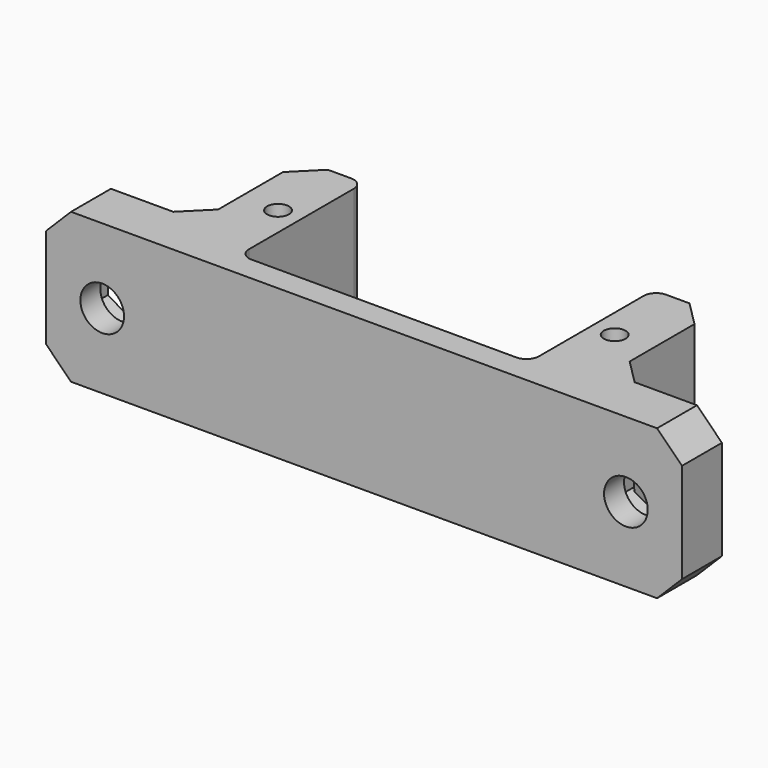
from build123d import *

# Parameters (mm, degrees)
F0_R         = 0.875
F1_DEPTH     = 12
F2_R         = 1.75
F3_DEPTH     = 4.001
F4_DEPTH     = 2
F5_T4_DEPTH  = 12
F5_T10_DEPTH = 12
F5_T16_DEPTH = 12
F5_T23_DEPTH = 12
F5_T29_DEPTH = 12
F5_T35_DEPTH = 12
F5_T41_DEPTH = 12
F5_T47_DEPTH = 12
F5_T54_DEPTH = 12
F5_T60_DEPTH = 12
F5_T63_DEPTH = 14.2867319519
F5_T65_DEPTH = 22.2867319519
F6_R         = 1


# Not quite as in the source:
# - a fillet or chamfer that OpenCascade refuses, or shapes differently, is made with other operations: its cross-section is extruded or revolved along the edge and cut away or added


with BuildPart() as f1:
    # F0 (on Top) → F1 (new body)
    with BuildSketch(Plane.XY):
        Polygon((16.5, -5.25), (11.625, -5.25), (-11.625, -5.25), (-16.5, -5.25), (-16.5, -7.25), (16.5, -7.25), align=None)
        Polygon((-11.625, -5.25), (-11.625, 7.25), (-16.5, 7.25), (-16.5, -3.25), (-16.5, -5.25), align=None)
        with Locations((-13.5, 1)):
            Circle(F0_R, mode=Mode.SUBTRACT)
        Polygon((16.5, -3.25), (16.5, 7.25), (11.625, 7.25), (11.625, -5.25), (16.5, -5.25), align=None)
        with Locations((13.5, 1)):
            Circle(F0_R, mode=Mode.SUBTRACT)
        Polygon((25.5, -3.25), (16.5, -3.25), (16.5, -5.25), (16.5, -7.25), (25.5, -7.25), align=None)
        Polygon((-16.5, -5.25), (-16.5, -3.25), (-25.5, -3.25), (-25.5, -7.25), (-16.5, -7.25), align=None)
    extrude(amount=F1_DEPTH)

    # F2 (on face) → F3 (cut, through all)
    with BuildSketch(Plane(origin=(0, -3.25, 0), x_dir=(-1, 0, 0), z_dir=(0, 1, 0))):
        with Locations((-21, 6)):
            Circle(F2_R)
        with Locations((21, 6)):
            Circle(F2_R)
    extrude(amount=-F3_DEPTH, mode=Mode.SUBTRACT)

    # F2 (on face) → F4 (cut)
    with BuildSketch(Plane(origin=(0, -3.25, 0), x_dir=(-1, 0, 0), z_dir=(0, 1, 0))):
        Polygon((-18.25, 4.4122867597), (-18.25, 7.5877132403), (-21, 9.1754264805), (-23.75, 7.5877132403), (-23.75, 4.4122867597), (-21, 2.8245735195), align=None)
        with Locations((-21, 6)):
            Circle(F2_R, mode=Mode.SUBTRACT)
        Polygon((21, 9.1754264805), (18.25, 7.5877132403), (18.25, 4.4122867597), (21, 2.8245735195), (23.75, 4.4122867597), (23.75, 7.5877132403), align=None)
        with Locations((21, 6)):
            Circle(F2_R, mode=Mode.SUBTRACT)
    extrude(amount=-F4_DEPTH, mode=Mode.SUBTRACT)

    # F5: chamfer of 2 on 8 edges, made by hand


with BuildPart() as f5_tool2:
    # F5_s3 → F5_t4 (new body)
    with BuildSketch(Plane.XY):
        Polygon((18.5, -3.25), (16.5, -1.25), (16.5, -3.25), align=None)
    extrude(amount=F5_T4_DEPTH)

    split(bisect_by=Plane.YZ.offset(18.25), keep=Keep.TOP)

    split(bisect_by=Plane(origin=(6.4730762114, 0, 11.2116968793), x_dir=(0, 1, 0), z_dir=(-0.5, 0, -0.8660254038)), keep=Keep.TOP)


with BuildPart() as f1_1:
    add(f1.part)

    # F5_t1: union F5_tool2
    add(f5_tool2.part)


with BuildPart() as f5_tool8:
    # F5_s9 → F5_t10 (new body)
    with BuildSketch(Plane.XY):
        Polygon((18.5, -3.25), (16.5, -1.25), (16.5, -3.25), align=None)
    extrude(amount=F5_T10_DEPTH)

    split(bisect_by=Plane.YZ.offset(18.25), keep=Keep.BOTTOM)

    split(bisect_by=Plane(origin=(6.4730762114, 0, 11.2116968793), x_dir=(0, 1, 0), z_dir=(-0.5, 0, -0.8660254038)), keep=Keep.TOP)


with BuildPart() as f1_2:
    add(f1_1.part)

    # F5_t7: union F5_tool8
    add(f5_tool8.part)


with BuildPart() as f5_tool14:
    # F5_s15 → F5_t16 (new body)
    with BuildSketch(Plane.XY):
        Polygon((18.5, -3.25), (16.5, -1.25), (16.5, -3.25), align=None)
    extrude(amount=F5_T16_DEPTH)

    split(bisect_by=Plane(origin=(1.2769237886, 0, -2.2116968793), x_dir=(0, 1, 0), z_dir=(0.5, 0, -0.8660254038)), keep=Keep.TOP)

    split(bisect_by=Plane.YZ.offset(18.25), keep=Keep.BOTTOM)

    split(bisect_by=Plane(origin=(6.4730762114, 0, 11.2116968793), x_dir=(0, 1, 0), z_dir=(0.5, 0, 0.8660254038)), keep=Keep.TOP)


with BuildPart() as f1_3:
    add(f1_2.part)

    # F5_t13: union F5_tool14
    add(f5_tool14.part)


with BuildPart() as f5_tool21:
    # F5_s22 → F5_t23 (new body)
    with BuildSketch(Plane.XY):
        Polygon((18.5, -3.25), (16.5, -1.25), (16.5, -3.25), align=None)
    extrude(amount=F5_T23_DEPTH)

    split(bisect_by=Plane(origin=(1.2769237886, 0, -2.2116968793), x_dir=(0, 1, 0), z_dir=(-0.5, 0, 0.8660254038)), keep=Keep.TOP)

    split(bisect_by=Plane.YZ.offset(18.25), keep=Keep.TOP)


with BuildPart() as f1_4:
    add(f1_3.part)

    # F5_t20: union F5_tool21
    add(f5_tool21.part)


with BuildPart() as f5_tool27:
    # F5_s28 → F5_t29 (new body)
    with BuildSketch(Plane.XY):
        Polygon((18.5, -3.25), (16.5, -1.25), (16.5, -3.25), align=None)
    extrude(amount=F5_T29_DEPTH)

    split(bisect_by=Plane(origin=(1.2769237886, 0, -2.2116968793), x_dir=(0, 1, 0), z_dir=(-0.5, 0, 0.8660254038)), keep=Keep.TOP)

    split(bisect_by=Plane.YZ.offset(18.25), keep=Keep.BOTTOM)


with BuildPart() as f1_5:
    add(f1_4.part)

    # F5_t26: union F5_tool27
    add(f5_tool27.part)


with BuildPart() as f5_tool33:
    # F5_s34 → F5_t35 (new body)
    with BuildSketch(Plane.XY):
        Polygon((-16.5, -1.25), (-18.5, -3.25), (-16.5, -3.25), align=None)
    extrude(amount=F5_T35_DEPTH)

    split(bisect_by=Plane(origin=(-6.4730762114, 0, 11.2116968793), x_dir=(0, 1, 0), z_dir=(0.5, 0, -0.8660254038)), keep=Keep.TOP)

    split(bisect_by=Plane.YZ.offset(-18.25), keep=Keep.TOP)


with BuildPart() as f1_6:
    add(f1_5.part)

    # F5_t32: union F5_tool33
    add(f5_tool33.part)


with BuildPart() as f5_tool39:
    # F5_s40 → F5_t41 (new body)
    with BuildSketch(Plane.XY):
        Polygon((-16.5, -1.25), (-18.5, -3.25), (-16.5, -3.25), align=None)
    extrude(amount=F5_T41_DEPTH)

    split(bisect_by=Plane(origin=(-6.4730762114, 0, 11.2116968793), x_dir=(0, 1, 0), z_dir=(0.5, 0, -0.8660254038)), keep=Keep.TOP)

    split(bisect_by=Plane.YZ.offset(-18.25), keep=Keep.BOTTOM)


with BuildPart() as f1_7:
    add(f1_6.part)

    # F5_t38: union F5_tool39
    add(f5_tool39.part)


with BuildPart() as f5_tool45:
    # F5_s46 → F5_t47 (new body)
    with BuildSketch(Plane.XY):
        Polygon((-16.5, -1.25), (-18.5, -3.25), (-16.5, -3.25), align=None)
    extrude(amount=F5_T47_DEPTH)

    split(bisect_by=Plane(origin=(-6.4730762114, 0, 11.2116968793), x_dir=(0, 1, 0), z_dir=(-0.5, 0, 0.8660254038)), keep=Keep.TOP)

    split(bisect_by=Plane.YZ.offset(-18.25), keep=Keep.TOP)

    split(bisect_by=Plane(origin=(-1.2769237886, 0, -2.2116968793), x_dir=(0, 1, 0), z_dir=(-0.5, 0, -0.8660254038)), keep=Keep.TOP)


with BuildPart() as f1_8:
    add(f1_7.part)

    # F5_t44: union F5_tool45
    add(f5_tool45.part)


with BuildPart() as f5_tool52:
    # F5_s53 → F5_t54 (new body)
    with BuildSketch(Plane.XY):
        Polygon((-16.5, -1.25), (-18.5, -3.25), (-16.5, -3.25), align=None)
    extrude(amount=F5_T54_DEPTH)

    split(bisect_by=Plane.YZ.offset(-18.25), keep=Keep.TOP)

    split(bisect_by=Plane(origin=(-1.2769237886, 0, -2.2116968793), x_dir=(0, 1, 0), z_dir=(0.5, 0, 0.8660254038)), keep=Keep.TOP)


with BuildPart() as f1_9:
    add(f1_8.part)

    # F5_t51: union F5_tool52
    add(f5_tool52.part)


with BuildPart() as f5_tool58:
    # F5_s59 → F5_t60 (new body)
    with BuildSketch(Plane.XY):
        Polygon((-16.5, -1.25), (-18.5, -3.25), (-16.5, -3.25), align=None)
    extrude(amount=F5_T60_DEPTH)

    split(bisect_by=Plane.YZ.offset(-18.25), keep=Keep.BOTTOM)

    split(bisect_by=Plane(origin=(-1.2769237886, 0, -2.2116968793), x_dir=(0, 1, 0), z_dir=(0.5, 0, 0.8660254038)), keep=Keep.TOP)


with BuildPart() as f1_10:
    add(f1_9.part)

    # F5_t57: union F5_tool58
    add(f5_tool58.part)

    # F5_s64 → F5_t63 (cut)
    with BuildSketch(Plane.XZ.offset(-1.8933659759)):
        Polygon((25.5, 2), (23.5, 0), (25.5, 0), align=None)
        Polygon((23.5, 12), (25.5, 10), (25.5, 12), align=None)
        Polygon((-25.5, 2), (-23.5, 0), (-25.5, 0), align=None)
        Polygon((-23.5, 12), (-25.5, 10), (-25.5, 12), align=None)
    extrude(amount=F5_T63_DEPTH, mode=Mode.SUBTRACT)

    # F5_s66 → F5_t65 (cut)
    with BuildSketch(Plane.XY.offset(-5.1433659759)):
        Polygon((14.5, 7.25), (16.5, 5.25), (16.5, 7.25), align=None)
        Polygon((-16.5, 5.25), (-14.5, 7.25), (-16.5, 7.25), align=None)
    extrude(amount=F5_T65_DEPTH, mode=Mode.SUBTRACT)

    # F6
    f6_edges = [f1_10.edges().sort_by_distance(p)[0] for p in [
        (-11.625, 7.25, 6),
        (11.625, 7.25, 6),
        (11.625, -5.25, 6),
        (-11.625, -5.25, 6),
    ]]
    fillet(f6_edges, radius=F6_R)


solid = f1_10.part
